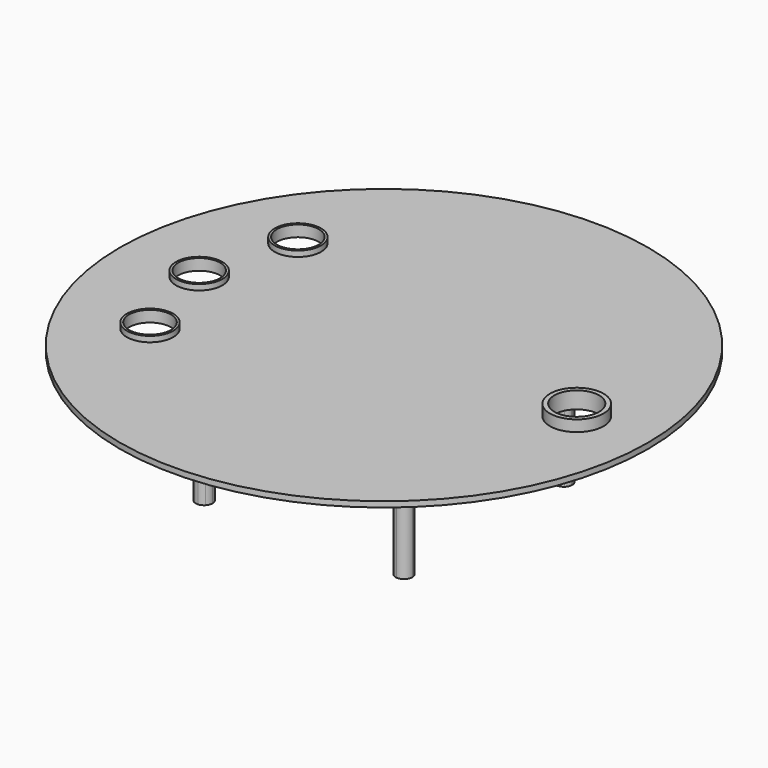
from build123d import *

# Parameters (mm, degrees)
F0_R     = 94.5
F0_R_2   = 8.3
F0_R_3   = 9.6
F1_DEPTH = 2
F0_R_4   = 7.5
F2_DEPTH = 4
F3_DEPTH = 2
F0_R_5   = 8
F4_DEPTH = 6
F5_DEPTH = 44


# Not quite as in the source:
# - a feature names something its author has since deleted; it is built from what else it names


with BuildPart() as f1:
    # F0 (on Top) → F1 (new body)
    with BuildSketch(Plane.XY):
        Circle(F0_R)
        with Locations((-57.2674702435, -33.0633893609)):
            Circle(F0_R_2, mode=Mode.SUBTRACT)
        with Locations((-66.1267787218, 0)):
            Circle(F0_R_2, mode=Mode.SUBTRACT)
        with Locations((-57.2674702435, 33.0633893609)):
            Circle(F0_R_2, mode=Mode.SUBTRACT)
        with BuildLine():
            ThreePointArc((38.7457430555, 35.5222910868), (48.9884210475, 19.0578165656), (52.5648720057, 0))
            ThreePointArc((52.5648720057, 0), (48.9884210475, -19.0578165656), (38.7457430555, -35.5222910868))
            ThreePointArc((38.7457430555, -35.5222910868), (38.7525078294, -35.6384400082), (38.7547638851, -35.7547638851))
            ThreePointArc((38.7547638851, -35.7547638851), (37.7922355542, -37.9567423585), (35.5222910868, -38.7457430555))
            ThreePointArc((35.5222910868, -38.7457430555), (0, -52.5648720057), (-35.5222910868, -38.7457430555))
            ThreePointArc((-35.5222910868, -38.7457430555), (-37.8760842286, -37.8760842286), (-38.7457430555, -35.5222910868))
            ThreePointArc((-38.7457430555, -35.5222910868), (-52.5648720057, 0), (-38.7457430555, 35.5222910868))
            ThreePointArc((-38.7457430555, 35.5222910868), (-37.8760842286, 37.8760842286), (-35.5222910868, 38.7457430555))
            ThreePointArc((-35.5222910868, 38.7457430555), (0, 52.5648720057), (35.5222910868, 38.7457430555))
            ThreePointArc((35.5222910868, 38.7457430555), (37.7922355542, 37.9567423585), (38.7547638851, 35.7547638851))
            ThreePointArc((38.7547638851, 35.7547638851), (38.7525078294, 35.6384400082), (38.7457430555, 35.5222910868))
        make_face(mode=Mode.SUBTRACT)
        with Locations((68.9690709114, 0)):
            Circle(F0_R_3, mode=Mode.SUBTRACT)
        with BuildLine():
            ThreePointArc((33.5714484549, 37.8122219605), (33.6334435415, 33.6334435415), (37.8122219605, 33.5714484549))
            ThreePointArc((37.8122219605, 33.5714484549), (35.7547638851, 35.7547638851), (33.5714484549, 37.8122219605))
        make_face()
        with BuildLine():
            ThreePointArc((-37.8122219605, 33.5714484549), (-38.4608914504, 34.459822342), (-38.7457430555, 35.5222910868))
            ThreePointArc((-38.7457430555, 35.5222910868), (-52.5648720057, 0), (-38.7457430555, -35.5222910868))
            ThreePointArc((-38.7457430555, -35.5222910868), (-38.4608914504, -34.459822342), (-37.8122219605, -33.5714484549))
            ThreePointArc((-37.8122219605, -33.5714484549), (-50.5648720057, 0), (-37.8122219605, 33.5714484549))
        make_face()
        with BuildLine():
            ThreePointArc((-35.5222910868, -38.7457430555), (0, -52.5648720057), (35.5222910868, -38.7457430555))
            ThreePointArc((35.5222910868, -38.7457430555), (34.459822342, -38.4608914504), (33.5714484549, -37.8122219605))
            ThreePointArc((33.5714484549, -37.8122219605), (0, -50.5648720057), (-33.5714484549, -37.8122219605))
            ThreePointArc((-33.5714484549, -37.8122219605), (-34.459822342, -38.4608914504), (-35.5222910868, -38.7457430555))
        make_face()
        with BuildLine():
            ThreePointArc((38.7457430555, -35.5222910868), (48.9884210475, -19.0578165656), (52.5648720057, 0))
            ThreePointArc((52.5648720057, 0), (48.9884210475, 19.0578165656), (38.7457430555, 35.5222910868))
            ThreePointArc((38.7457430555, 35.5222910868), (38.4608914504, 34.459822342), (37.8122219605, 33.5714484549))
            ThreePointArc((37.8122219605, 33.5714484549), (47.2693158647, 17.9560034148), (50.5648720057, 0))
            ThreePointArc((50.5648720057, 0), (47.2693158647, -17.9560034148), (37.8122219605, -33.5714484549))
            ThreePointArc((37.8122219605, -33.5714484549), (38.4608914504, -34.459822342), (38.7457430555, -35.5222910868))
        make_face()
        with BuildLine():
            ThreePointArc((33.5714484549, 37.8122219605), (34.459822342, 38.4608914504), (35.5222910868, 38.7457430555))
            ThreePointArc((35.5222910868, 38.7457430555), (0, 52.5648720057), (-35.5222910868, 38.7457430555))
            ThreePointArc((-35.5222910868, 38.7457430555), (-34.459822342, 38.4608914504), (-33.5714484549, 37.8122219605))
            ThreePointArc((-33.5714484549, 37.8122219605), (0, 50.5648720057), (33.5714484549, 37.8122219605))
        make_face()
        with BuildLine():
            ThreePointArc((33.5714484549, -37.8122219605), (35.7547638851, -35.7547638851), (37.8122219605, -33.5714484549))
            ThreePointArc((37.8122219605, -33.5714484549), (33.6334435415, -33.6334435415), (33.5714484549, -37.8122219605))
        make_face()
        with BuildLine():
            ThreePointArc((35.5222910868, -38.7457430555), (37.1689774474, -37.1689774474), (38.7457430555, -35.5222910868))
            ThreePointArc((38.7457430555, -35.5222910868), (38.4608914504, -34.459822342), (37.8122219605, -33.5714484549))
            ThreePointArc((37.8122219605, -33.5714484549), (35.7547638851, -35.7547638851), (33.5714484549, -37.8122219605))
            ThreePointArc((33.5714484549, -37.8122219605), (34.459822342, -38.4608914504), (35.5222910868, -38.7457430555))
        make_face()
        with BuildLine():
            ThreePointArc((38.7547638851, -35.7547638851), (38.7525078294, -35.6384400082), (38.7457430555, -35.5222910868))
            ThreePointArc((38.7457430555, -35.5222910868), (37.1689774474, -37.1689774474), (35.5222910868, -38.7457430555))
            ThreePointArc((35.5222910868, -38.7457430555), (37.7922355542, -37.9567423585), (38.7547638851, -35.7547638851))
        make_face()
        with BuildLine():
            ThreePointArc((50.5648720057, 0), (47.2693158647, 17.9560034148), (37.8122219605, 33.5714484549))
            ThreePointArc((37.8122219605, 33.5714484549), (33.6334435415, 33.6334435415), (33.5714484549, 37.8122219605))
            ThreePointArc((33.5714484549, 37.8122219605), (0, 50.5648720057), (-33.5714484549, 37.8122219605))
            ThreePointArc((-33.5714484549, 37.8122219605), (-32.9664000018, 36.8615731978), (-32.7547638851, 35.7547638851))
            ThreePointArc((-32.7547638851, 35.7547638851), (-34.5657252453, 33.0004605043), (-37.8122219605, 33.5714484549))
            ThreePointArc((-37.8122219605, 33.5714484549), (-50.5648720057, 0), (-37.8122219605, -33.5714484549))
            ThreePointArc((-37.8122219605, -33.5714484549), (-34.5657252453, -33.0004605043), (-32.7547638851, -35.7547638851))
            ThreePointArc((-32.7547638851, -35.7547638851), (-32.9664000018, -36.8615731978), (-33.5714484549, -37.8122219605))
            ThreePointArc((-33.5714484549, -37.8122219605), (0, -50.5648720057), (33.5714484549, -37.8122219605))
            ThreePointArc((33.5714484549, -37.8122219605), (33.6334435415, -33.6334435415), (37.8122219605, -33.5714484549))
            ThreePointArc((37.8122219605, -33.5714484549), (47.2693158647, -17.9560034148), (50.5648720057, 0))
        make_face()
        with BuildLine():
            ThreePointArc((37.8122219605, 33.5714484549), (38.4608914504, 34.459822342), (38.7457430555, 35.5222910868))
            ThreePointArc((38.7457430555, 35.5222910868), (37.1689774474, 37.1689774474), (35.5222910868, 38.7457430555))
            ThreePointArc((35.5222910868, 38.7457430555), (34.459822342, 38.4608914504), (33.5714484549, 37.8122219605))
            ThreePointArc((33.5714484549, 37.8122219605), (35.7547638851, 35.7547638851), (37.8122219605, 33.5714484549))
        make_face()
        with BuildLine():
            ThreePointArc((35.5222910868, 38.7457430555), (37.1689774474, 37.1689774474), (38.7457430555, 35.5222910868))
            ThreePointArc((38.7457430555, 35.5222910868), (38.7525078294, 35.6384400082), (38.7547638851, 35.7547638851))
            ThreePointArc((38.7547638851, 35.7547638851), (37.7922355542, 37.9567423585), (35.5222910868, 38.7457430555))
        make_face()
        with BuildLine():
            ThreePointArc((-38.7457430555, 35.5222910868), (-37.1689774474, 37.1689774474), (-35.5222910868, 38.7457430555))
            ThreePointArc((-35.5222910868, 38.7457430555), (-37.8760842286, 37.8760842286), (-38.7457430555, 35.5222910868))
        make_face()
        with BuildLine():
            ThreePointArc((-33.5714484549, 37.8122219605), (-34.459822342, 38.4608914504), (-35.5222910868, 38.7457430555))
            ThreePointArc((-35.5222910868, 38.7457430555), (-37.1689774474, 37.1689774474), (-38.7457430555, 35.5222910868))
            ThreePointArc((-38.7457430555, 35.5222910868), (-38.4608914504, 34.459822342), (-37.8122219605, 33.5714484549))
            ThreePointArc((-37.8122219605, 33.5714484549), (-35.7547638851, 35.7547638851), (-33.5714484549, 37.8122219605))
        make_face()
        with BuildLine():
            ThreePointArc((-32.7547638851, 35.7547638851), (-32.9664000018, 36.8615731978), (-33.5714484549, 37.8122219605))
            ThreePointArc((-33.5714484549, 37.8122219605), (-35.7547638851, 35.7547638851), (-37.8122219605, 33.5714484549))
            ThreePointArc((-37.8122219605, 33.5714484549), (-34.5657252453, 33.0004605043), (-32.7547638851, 35.7547638851))
        make_face()
        with BuildLine():
            ThreePointArc((-38.7457430555, -35.5222910868), (-37.8760842286, -37.8760842286), (-35.5222910868, -38.7457430555))
            ThreePointArc((-35.5222910868, -38.7457430555), (-37.1689774474, -37.1689774474), (-38.7457430555, -35.5222910868))
        make_face()
        with BuildLine():
            ThreePointArc((-38.7457430555, -35.5222910868), (-37.1689774474, -37.1689774474), (-35.5222910868, -38.7457430555))
            ThreePointArc((-35.5222910868, -38.7457430555), (-34.459822342, -38.4608914504), (-33.5714484549, -37.8122219605))
            ThreePointArc((-33.5714484549, -37.8122219605), (-35.7547638851, -35.7547638851), (-37.8122219605, -33.5714484549))
            ThreePointArc((-37.8122219605, -33.5714484549), (-38.4608914504, -34.459822342), (-38.7457430555, -35.5222910868))
        make_face()
        with BuildLine():
            ThreePointArc((-37.8122219605, -33.5714484549), (-35.7547638851, -35.7547638851), (-33.5714484549, -37.8122219605))
            ThreePointArc((-33.5714484549, -37.8122219605), (-32.9664000018, -36.8615731978), (-32.7547638851, -35.7547638851))
            ThreePointArc((-32.7547638851, -35.7547638851), (-34.5657252453, -33.0004605043), (-37.8122219605, -33.5714484549))
        make_face()
    extrude(amount=F1_DEPTH)

    # F0 (on Top) → F2 (join)
    with BuildSketch(Plane.XY):
        with Locations((-57.2674702435, 33.0633893609)):
            Circle(F0_R_2)
        with Locations((-57.2674702435, 33.0633893609)):
            Circle(F0_R_4, mode=Mode.SUBTRACT)
        with Locations((-66.1267787218, 0)):
            Circle(F0_R_2)
        with Locations((-66.1267787218, 0)):
            Circle(F0_R_4, mode=Mode.SUBTRACT)
        with Locations((-57.2674702435, -33.0633893609)):
            Circle(F0_R_2)
        with Locations((-57.2674702435, -33.0633893609)):
            Circle(F0_R_4, mode=Mode.SUBTRACT)
    extrude(amount=F2_DEPTH)

    # F0 (on Top) → F3 (join)
    with BuildSketch(Plane.XY):
        with BuildLine():
            ThreePointArc((-37.8122219605, 33.5714484549), (-38.4608914504, 34.459822342), (-38.7457430555, 35.5222910868))
            ThreePointArc((-38.7457430555, 35.5222910868), (-52.5648720057, 0), (-38.7457430555, -35.5222910868))
            ThreePointArc((-38.7457430555, -35.5222910868), (-38.4608914504, -34.459822342), (-37.8122219605, -33.5714484549))
            ThreePointArc((-37.8122219605, -33.5714484549), (-50.5648720057, 0), (-37.8122219605, 33.5714484549))
        make_face()
        with BuildLine():
            ThreePointArc((-35.5222910868, -38.7457430555), (0, -52.5648720057), (35.5222910868, -38.7457430555))
            ThreePointArc((35.5222910868, -38.7457430555), (34.459822342, -38.4608914504), (33.5714484549, -37.8122219605))
            ThreePointArc((33.5714484549, -37.8122219605), (0, -50.5648720057), (-33.5714484549, -37.8122219605))
            ThreePointArc((-33.5714484549, -37.8122219605), (-34.459822342, -38.4608914504), (-35.5222910868, -38.7457430555))
        make_face()
        with BuildLine():
            ThreePointArc((38.7457430555, -35.5222910868), (48.9884210475, -19.0578165656), (52.5648720057, 0))
            ThreePointArc((52.5648720057, 0), (48.9884210475, 19.0578165656), (38.7457430555, 35.5222910868))
            ThreePointArc((38.7457430555, 35.5222910868), (38.4608914504, 34.459822342), (37.8122219605, 33.5714484549))
            ThreePointArc((37.8122219605, 33.5714484549), (47.2693158647, 17.9560034148), (50.5648720057, 0))
            ThreePointArc((50.5648720057, 0), (47.2693158647, -17.9560034148), (37.8122219605, -33.5714484549))
            ThreePointArc((37.8122219605, -33.5714484549), (38.4608914504, -34.459822342), (38.7457430555, -35.5222910868))
        make_face()
        with BuildLine():
            ThreePointArc((33.5714484549, 37.8122219605), (34.459822342, 38.4608914504), (35.5222910868, 38.7457430555))
            ThreePointArc((35.5222910868, 38.7457430555), (0, 52.5648720057), (-35.5222910868, 38.7457430555))
            ThreePointArc((-35.5222910868, 38.7457430555), (-34.459822342, 38.4608914504), (-33.5714484549, 37.8122219605))
            ThreePointArc((-33.5714484549, 37.8122219605), (0, 50.5648720057), (33.5714484549, 37.8122219605))
        make_face()
    extrude(amount=-F3_DEPTH)

    # F0 (on Top) → F4 (join)
    with BuildSketch(Plane.XY):
        with Locations((68.9690709114, 0)):
            Circle(F0_R_3)
        with Locations((68.9690709114, 0)):
            Circle(F0_R_5, mode=Mode.SUBTRACT)
    extrude(amount=F4_DEPTH)

    # F0 (on Top) → F5 (join)
    with BuildSketch(Plane.XY):
        with BuildLine():
            ThreePointArc((37.8122219605, 33.5714484549), (38.4608914504, 34.459822342), (38.7457430555, 35.5222910868))
            ThreePointArc((38.7457430555, 35.5222910868), (37.1689774474, 37.1689774474), (35.5222910868, 38.7457430555))
            ThreePointArc((35.5222910868, 38.7457430555), (34.459822342, 38.4608914504), (33.5714484549, 37.8122219605))
            ThreePointArc((33.5714484549, 37.8122219605), (35.7547638851, 35.7547638851), (37.8122219605, 33.5714484549))
        make_face()
        with BuildLine():
            ThreePointArc((35.5222910868, 38.7457430555), (37.1689774474, 37.1689774474), (38.7457430555, 35.5222910868))
            ThreePointArc((38.7457430555, 35.5222910868), (38.7525078294, 35.6384400082), (38.7547638851, 35.7547638851))
            ThreePointArc((38.7547638851, 35.7547638851), (37.7922355542, 37.9567423585), (35.5222910868, 38.7457430555))
        make_face()
        with BuildLine():
            ThreePointArc((38.7547638851, -35.7547638851), (38.7525078294, -35.6384400082), (38.7457430555, -35.5222910868))
            ThreePointArc((38.7457430555, -35.5222910868), (37.1689774474, -37.1689774474), (35.5222910868, -38.7457430555))
            ThreePointArc((35.5222910868, -38.7457430555), (37.7922355542, -37.9567423585), (38.7547638851, -35.7547638851))
        make_face()
        with BuildLine():
            ThreePointArc((35.5222910868, -38.7457430555), (37.1689774474, -37.1689774474), (38.7457430555, -35.5222910868))
            ThreePointArc((38.7457430555, -35.5222910868), (38.4608914504, -34.459822342), (37.8122219605, -33.5714484549))
            ThreePointArc((37.8122219605, -33.5714484549), (35.7547638851, -35.7547638851), (33.5714484549, -37.8122219605))
            ThreePointArc((33.5714484549, -37.8122219605), (34.459822342, -38.4608914504), (35.5222910868, -38.7457430555))
        make_face()
        with BuildLine():
            ThreePointArc((33.5714484549, 37.8122219605), (33.6334435415, 33.6334435415), (37.8122219605, 33.5714484549))
            ThreePointArc((37.8122219605, 33.5714484549), (35.7547638851, 35.7547638851), (33.5714484549, 37.8122219605))
        make_face()
        with BuildLine():
            ThreePointArc((33.5714484549, -37.8122219605), (35.7547638851, -35.7547638851), (37.8122219605, -33.5714484549))
            ThreePointArc((37.8122219605, -33.5714484549), (33.6334435415, -33.6334435415), (33.5714484549, -37.8122219605))
        make_face()
        with BuildLine():
            ThreePointArc((-33.5714484549, 37.8122219605), (-34.459822342, 38.4608914504), (-35.5222910868, 38.7457430555))
            ThreePointArc((-35.5222910868, 38.7457430555), (-37.1689774474, 37.1689774474), (-38.7457430555, 35.5222910868))
            ThreePointArc((-38.7457430555, 35.5222910868), (-38.4608914504, 34.459822342), (-37.8122219605, 33.5714484549))
            ThreePointArc((-37.8122219605, 33.5714484549), (-35.7547638851, 35.7547638851), (-33.5714484549, 37.8122219605))
        make_face()
        with BuildLine():
            ThreePointArc((-38.7457430555, 35.5222910868), (-37.1689774474, 37.1689774474), (-35.5222910868, 38.7457430555))
            ThreePointArc((-35.5222910868, 38.7457430555), (-37.8760842286, 37.8760842286), (-38.7457430555, 35.5222910868))
        make_face()
        with BuildLine():
            ThreePointArc((-38.7457430555, -35.5222910868), (-37.8760842286, -37.8760842286), (-35.5222910868, -38.7457430555))
            ThreePointArc((-35.5222910868, -38.7457430555), (-37.1689774474, -37.1689774474), (-38.7457430555, -35.5222910868))
        make_face()
        with BuildLine():
            ThreePointArc((-38.7457430555, -35.5222910868), (-37.1689774474, -37.1689774474), (-35.5222910868, -38.7457430555))
            ThreePointArc((-35.5222910868, -38.7457430555), (-34.459822342, -38.4608914504), (-33.5714484549, -37.8122219605))
            ThreePointArc((-33.5714484549, -37.8122219605), (-35.7547638851, -35.7547638851), (-37.8122219605, -33.5714484549))
            ThreePointArc((-37.8122219605, -33.5714484549), (-38.4608914504, -34.459822342), (-38.7457430555, -35.5222910868))
        make_face()
        with BuildLine():
            ThreePointArc((-32.7547638851, 35.7547638851), (-32.9664000018, 36.8615731978), (-33.5714484549, 37.8122219605))
            ThreePointArc((-33.5714484549, 37.8122219605), (-35.7547638851, 35.7547638851), (-37.8122219605, 33.5714484549))
            ThreePointArc((-37.8122219605, 33.5714484549), (-34.5657252453, 33.0004605043), (-32.7547638851, 35.7547638851))
        make_face()
        with BuildLine():
            ThreePointArc((-37.8122219605, -33.5714484549), (-35.7547638851, -35.7547638851), (-33.5714484549, -37.8122219605))
            ThreePointArc((-33.5714484549, -37.8122219605), (-32.9664000018, -36.8615731978), (-32.7547638851, -35.7547638851))
            ThreePointArc((-32.7547638851, -35.7547638851), (-34.5657252453, -33.0004605043), (-37.8122219605, -33.5714484549))
        make_face()
    extrude(amount=-F5_DEPTH)


solid = f1.part
